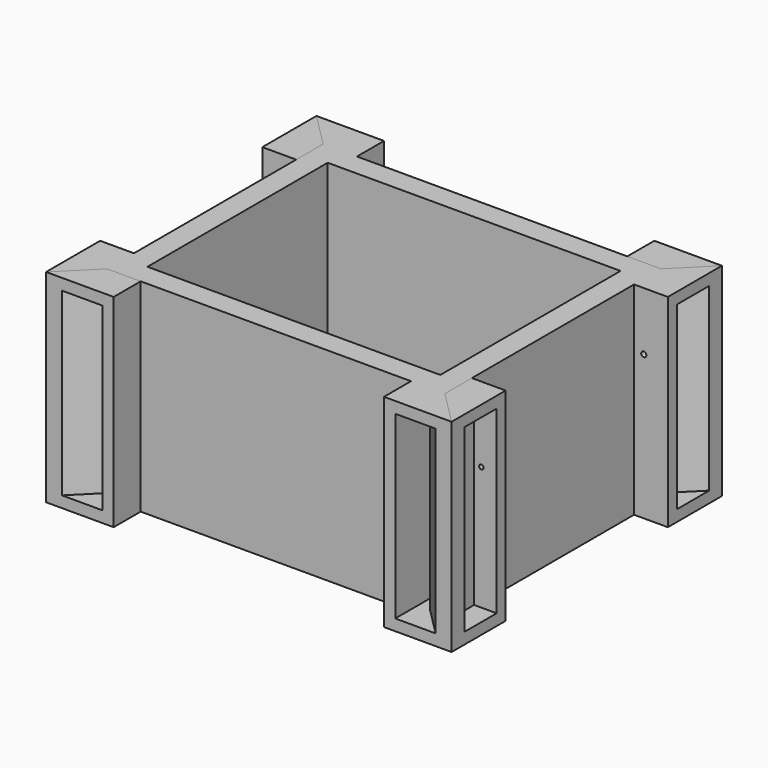
from build123d import *

# Parameters (mm, degrees)
F1_DEPTH      = 45
F2_DEPTH      = 45
F3_DEPTH      = 3
F4_T          = -2.5
F4_2_T        = -2.5
F5_DEPTH      = 45
F6_T          = 2.5
F6_T3_DEPTH   = 50
F6_2_T        = -2.5
F6_3_T        = -2.5
F7_R          = 0.4177450637
F8_DEPTH      = 3.6
F10_R         = 0.4781822673
F11_DEPTH     = 3.7
F12_R         = 0.5705514109
F13_DEPTH     = 3.5
F14_R         = 0.4924702409
F15_DEPTH     = 4.5
F16_TEXT_SIZE = 9.6982733036
F17_DEPTH     = 2


# Not quite as in the source:
# - a shell that OpenCascade refuses in one call is made with other operations: the cavity is built on its own and cut out
# - a feature names something its author has since deleted; it is built from what else it names
# - Text() gives the source's letters only with a copy of the font that has no kerning and outlines rounded to 1/6400 em; it was checked with that copy


with BuildPart() as f1:
    # F0 (on Top) → F1 (new body)
    with BuildSketch(Plane.XY):
        Polygon((37.5, 22.5), (37.5, 30), (30, 30), (-30, 30), (-37.5, 30), (-37.5, 22.5), (-37.5, -22.5), (-37.5, -30), (-30, -30), (30, -30), (37.5, -30), (37.5, -22.5), align=None)
        Polygon((-32.5, 25), (32.5, 25), (32.5, -25), (-32.5, -25), (-32.5, 24.8922383785), align=None, mode=Mode.SUBTRACT)
    extrude(amount=F1_DEPTH)

    # F0 (on Top) → F5 (join)
    with BuildSketch(Plane.XY):
        Polygon((-37.5, 30), (-30, 30), (-30, 37.5), (-45, 37.5), align=None)
        Polygon((45, 37.5), (37.5, 30), (37.5, 22.5), (45, 22.5), align=None)
        Polygon((45, -37.5), (37.5, -30), (30, -30), (30, -37.5), align=None)
        Polygon((-37.5, -30), (-37.5, -22.5), (-45, -22.5), (-45, -37.5), align=None)
    extrude(amount=F5_DEPTH)

    # F6: shell of thickness 2.5, made by hand


with BuildPart() as f2:
    # F0 (on Top) → F2 (new body)
    with BuildSketch(Plane.XY):
        Polygon((-30, -37.5), (-30, -30), (-37.5, -30), (-45, -37.5), align=None)
    extrude(amount=F2_DEPTH)

    # F4
    f4_openings = [f2.faces().sort_by_distance(p)[0] for p in [
        (-37.5, -37.5, 22.5),
    ]]
    offset(amount=F4_T, openings=f4_openings)


with BuildPart() as f2b:
    # F0 (on Top) → F2, piece 2 (new body)
    with BuildSketch(Plane.XY):
        Polygon((-37.5, 22.5), (-37.5, 30), (-45, 37.5), (-45, 22.5), align=None)
    extrude(amount=F2_DEPTH)

    # F4#2
    f4_2_openings = [f2b.faces().sort_by_distance(p)[0] for p in [
        (-45, 30, 22.5),
    ]]
    offset(amount=F4_2_T, openings=f4_2_openings)

    # F7 (on face) → F8 (cut)
    with BuildSketch(Plane.XZ.offset(-22.5)):
        with Locations((-41.25, 31.6409021616)):
            Circle(F7_R)
    extrude(amount=-F8_DEPTH, mode=Mode.SUBTRACT)


with BuildPart() as f2c:
    # F0 (on Top) → F2, piece 3 (new body)
    with BuildSketch(Plane.XY):
        Polygon((30, 30), (37.5, 30), (45, 37.5), (30, 37.5), align=None)
    extrude(amount=F2_DEPTH)

    # F6#3
    f6_3_openings = [f2c.faces().sort_by_distance(p)[0] for p in [
        (37.5, 37.5, 22.5),
    ]]
    offset(amount=F6_3_T, openings=f6_3_openings)


with BuildPart() as f2d:
    # F0 (on Top) → F2, piece 4 (new body)
    with BuildSketch(Plane.XY):
        Polygon((45, -22.5), (37.5, -22.5), (37.5, -30), (45, -37.5), align=None)
    extrude(amount=F2_DEPTH)

    # F6#2
    f6_2_openings = [f2d.faces().sort_by_distance(p)[0] for p in [
        (45, -30, 22.5),
    ]]
    offset(amount=F6_2_T, openings=f6_2_openings)

    # F14 (on face) → F15 (cut)
    with BuildSketch(Plane(origin=(0, -22.5, 0), x_dir=(-1, 0, 0), z_dir=(0, 1, 0))):
        with Locations((-41.6103377938, 29.9775898457)):
            Circle(F14_R)
    extrude(amount=-F15_DEPTH, mode=Mode.SUBTRACT)


with BuildPart() as f3:
    # F0 (on Top) → F3 (new body)
    with BuildSketch(Plane.XY):
        Polygon((32.5, -25), (32.5, 25), (-32.5, 25), (-32.5, 24.8922383785), (-32.5, -25), align=None)
    extrude(amount=F3_DEPTH)


with BuildPart() as f6_core1:
    # F6_t2: copy of F1
    add(f1.part)

    # the walls: a layer under each face that stays
    f6_faces = [f6_core1.faces().sort_by_distance(p)[0] for p in [
        (37.5, -3.75, 22.5),
        (41.25, 22.5, 22.5),
        (-38.5714285714, 32.1428571429, 45),
        (41.25, -33.75, 22.5),
        (-38.5714285714, 32.1428571429, 0),
        (3.75, 30, 22.5),
        (-37.5, 3.75, 22.5),
        (-3.75, -30, 22.5),
        (0, 25, 22.5),
        (32.5, 0, 22.5),
        (0, -25, 22.5),
        (-32.5, 0, 22.5),
        (41.25, 33.75, 22.5),
        (-30, 33.75, 22.5),
        (-41.25, 33.75, 22.5),
        (-41.25, -22.5, 22.5),
        (-41.25, -33.75, 22.5),
        (30, -33.75, 22.5),
    ]]
    thicken(f6_faces, amount=-F6_T, mode=Mode.SUBTRACT)

    # F6_s4 → F6_t3 (cut)
    with BuildSketch(Plane.XY.offset(-2.5)):
        Polygon((37.525, 22.475), (35, 22.5), (35, 25), (37.5, 25), align=None)
        Polygon((37.5426776695, -29.9823223305), (35, -30), (35, -31.0355339059), (35.732233047, -31.767766953), align=None)
        Polygon((-29.975, 30.025), (-30, 27.5), (-32.5, 27.5), (-32.5, 30), align=None)
        Polygon((37.4823223305, 30.0426776695), (37.5, 27.5), (38.5355339059, 27.5), (39.267766953, 28.232233047), align=None)
        Polygon((-37.525, -22.475), (-35, -22.5), (-35, -25), (-37.5, -25), align=None)
        Polygon((-37.5426776695, 29.9823223305), (-35, 30), (-35, 31.0355339059), (-35.732233047, 31.767766953), align=None)
        Polygon((29.975, -30.025), (30, -27.5), (32.5, -27.5), (32.5, -30), align=None)
        Polygon((-37.4823223305, -30.0426776695), (-37.5, -27.5), (-38.5355339059, -27.5), (-39.267766953, -28.232233047), align=None)
        Polygon((-32.475, 24.975), (-32.5, 27.5), (-35, 27.5), (-35, 25), align=None)
        Polygon((32.475, 24.975), (32.5, 27.5), (35, 27.5), (35, 25), align=None)
        Polygon((32.475, -24.975), (35, -25), (35, -27.5), (32.5, -27.5), align=None)
        Polygon((-32.475, -24.975), (-32.5, -27.5), (-35, -27.5), (-35, -25), align=None)
    extrude(amount=F6_T3_DEPTH, mode=Mode.SUBTRACT)


with BuildPart() as f1_1:
    add(f1.part)

    # what is left inside the walls is the cavity
    f6_cavity = [f6_core1.part.solids().sort_by_distance(p)[0] for p in [
        (32.525, -32.5, 29.166667),
        (40, 25.025, 29.166667),
        (-40, -25.025, 29.166667),
        (-32.525, 32.5, 29.166667),
    ]]
    add(f6_cavity, mode=Mode.SUBTRACT)

    # F10 (on face) → F11 (cut)
    with BuildSketch(Plane(origin=(0, -22.5, 0), x_dir=(-1, 0, 0), z_dir=(0, 1, 0))):
        with Locations((39.2241925001, 30.3633082658)):
            Circle(F10_R)
    extrude(amount=-F11_DEPTH, mode=Mode.SUBTRACT)

    # F12 (on face) → F13 (cut)
    with BuildSketch(Plane.XZ.offset(-22.5)):
        with Locations((39.6584272385, 32.0557616651)):
            Circle(F12_R)
    extrude(amount=-F13_DEPTH, mode=Mode.SUBTRACT)

    # F16 (on face) → F17 (join)
    with BuildSketch(Plane(origin=(0, 30, 0), x_dir=(-1, 0, 0), z_dir=(0, 1, 0))):
        with Locations((-21.8871365068, 32.5666517019)):
            Text('dylan', F16_TEXT_SIZE, font='Open Sans', font_style=FontStyle.BOLD, text_align=(TextAlign.LEFT, TextAlign.BOTTOM))
        with Locations((-21.8871365068, 19.377000009)):
            Text("pratt's", F16_TEXT_SIZE, font='Open Sans', font_style=FontStyle.BOLD, text_align=(TextAlign.LEFT, TextAlign.BOTTOM))
        with Locations((-21.8871365068, 6.1873483161)):
            Text('box', F16_TEXT_SIZE, font='Open Sans', font_style=FontStyle.BOLD, text_align=(TextAlign.LEFT, TextAlign.BOTTOM))
    extrude(amount=F17_DEPTH)


solid = Compound([f2.part, f2b.part, f2c.part, f2d.part, f3.part, f1_1.part])
